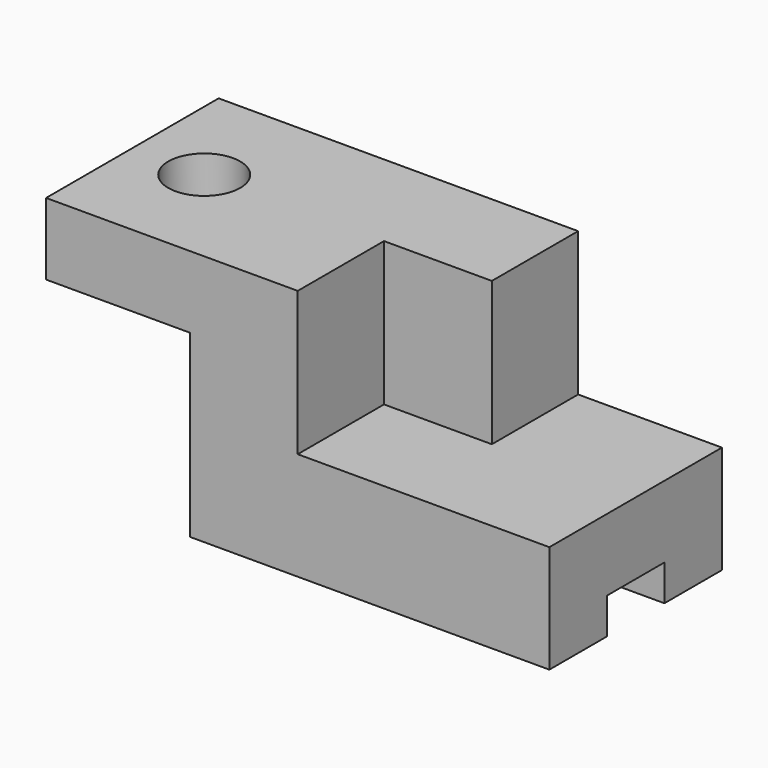
from build123d import *

# Parameters (mm, degrees)
F0_W     = 50
F0_H     = 30
F1_DEPTH = 15
F2_W     = 10
F2_H     = 5
F3_DEPTH = 50
F5_DEPTH = 10
F6_W     = 20
F6_H     = 30
F7_DEPTH = 10
F8_R     = 5
F9_DEPTH = 25


with BuildPart() as f1:
    # F0 (on Top) → F1 (new body)
    with BuildSketch(Plane.XY):
        with Locations((-0.216518305, -0.4101539962)):
            Rectangle(F0_W, F0_H)
    extrude(amount=F1_DEPTH)

    # F2 (on face) → F3 (cut)
    with BuildSketch(Plane.YZ.offset(24.783481695)):
        with Locations((-0.4101539962, 2.5)):
            Rectangle(F2_W, F2_H)
    extrude(amount=-F3_DEPTH, mode=Mode.SUBTRACT)

    # F4 (on face) → F5 (join)
    with BuildSketch(Plane.XY.offset(15)):
        Polygon((-25.216518305, 14.5898460038), (-25.216518305, -15.4101539962), (-10.216518305, -15.4101539962), (-10.216518305, -0.4101539962), (4.783481695, -0.4101539962), (4.783481695, 14.5898460038), align=None)
    extrude(amount=F5_DEPTH)

    # F6 (on face) → F7 (join)
    with BuildSketch(Plane.XY.offset(25)):
        with Locations((-35.216518305, -0.4101539962)):
            Rectangle(F6_W, F6_H)
        Polygon((-25.216518305, 14.5898460038), (-25.216518305, -15.4101539962), (-10.216518305, -15.4101539962), (-10.216518305, -0.4101539962), (4.783481695, -0.4101539962), (4.783481695, 14.5898460038), align=None)
    extrude(amount=F7_DEPTH)

    # F8 (on face) → F9 (cut)
    with BuildSketch(Plane.XY.offset(35)):
        with Locations((-35.216518305, -0.4101539962)):
            Circle(F8_R)
    extrude(amount=-F9_DEPTH, mode=Mode.SUBTRACT)


solid = f1.part
